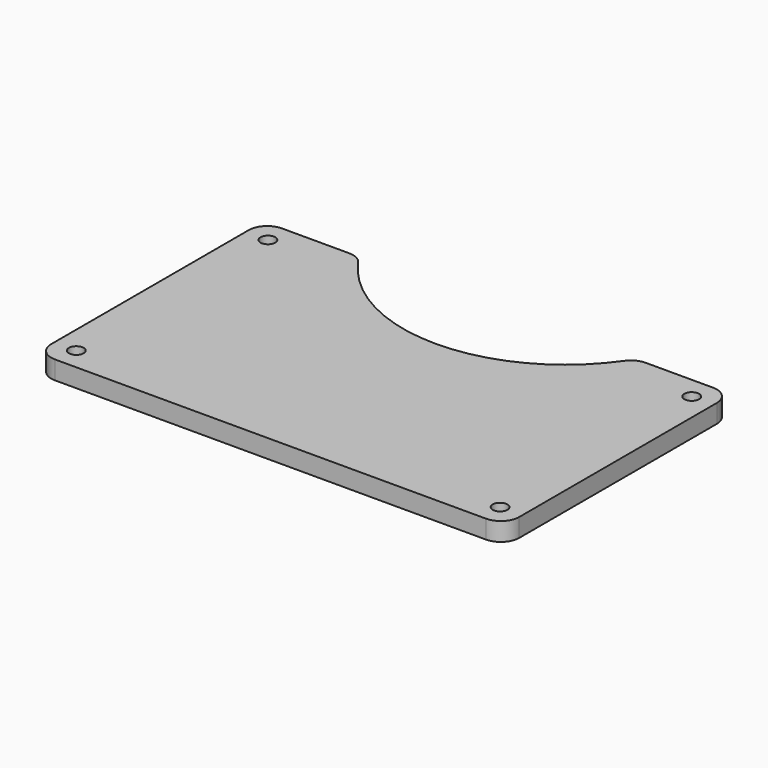
from build123d import *

# Parameters (mm, degrees)
F0_R     = 2
F1_DEPTH = 5
F2_R     = 3
F3_DEPTH = 0.6
F5_DEPTH = 2
F6_R     = 10
F7_R     = 2.5


with BuildPart() as f1:
    # F0 (on Top) → F1 (new body)
    with BuildSketch(Plane.XY):
        with BuildLine():
            Line((-58.5, -38.5), (58.5, -38.5))
            ThreePointArc((58.5, -38.5), (62.0355339059, -37.0355339059), (63.5, -33.5))
            Line((63.5, -33.5), (63.5, 33.5))
            ThreePointArc((63.5, 33.5), (62.0355339059, 37.0355339059), (58.5, 38.5))
            Line((58.5, 38.5), (40.2026118555, 38.5))
            ThreePointArc((40.2026118555, 38.5), (37.8876397432, 37.9318059659), (36.0988089683, 36.3563616478))
            ThreePointArc((36.0988089683, 36.3563616478), (0, 17.5), (-36.0988089683, 36.3563616478))
            ThreePointArc((-36.0988089683, 36.3563616478), (-37.8876397432, 37.9318059659), (-40.2026118555, 38.5))
            Line((-40.2026118555, 38.5), (-58.5, 38.5))
            ThreePointArc((-58.5, 38.5), (-62.0355339059, 37.0355339059), (-63.5, 33.5))
            Line((-63.5, 33.5), (-63.5, -33.5))
            ThreePointArc((-63.5, -33.5), (-62.0355339059, -37.0355339059), (-58.5, -38.5))
        make_face()
        with Locations((-57.5, -32.5)):
            Circle(F0_R, mode=Mode.SUBTRACT)
        with Locations((57.5, -32.5)):
            Circle(F0_R, mode=Mode.SUBTRACT)
        with Locations((-57.5, 32.5)):
            Circle(F0_R, mode=Mode.SUBTRACT)
        with Locations((57.5, 32.5)):
            Circle(F0_R, mode=Mode.SUBTRACT)
    extrude(amount=F1_DEPTH)

    # F2 (on face) → F3 (cut)
    with BuildSketch(Plane(origin=(0, 0, 0), x_dir=(1, 0, 0), z_dir=(0, 0, -1))):
        with Locations((-57.5, 32.5)):
            Circle(F2_R)
        with Locations((57.5, 32.5)):
            Circle(F2_R)
        with Locations((57.5, -32.5)):
            Circle(F2_R)
        with Locations((-57.5, -32.5)):
            Circle(F2_R)
    extrude(amount=-F3_DEPTH, mode=Mode.SUBTRACT)

    # F4 (on face) → F5 (cut)
    with BuildSketch(Plane(origin=(0, 0, 0), x_dir=(1, 0, 0), z_dir=(0, 0, -1))):
        Polygon((-8.542372966, 0), (-57.5000000613, 26.5), (-57.5, -26.5), align=None)
        Polygon((-4.0665, 32.5000000613), (-51.5, 32.5000000613), (-4.0665, 6.8249862876), align=None)
        Polygon((51.5, 32.5000000613), (4.0665, 32.5000000613), (4.0665, 6.8249862876), align=None)
        Polygon((57.5000000613, 26.5), (8.542372966, 0), (57.5000000613, -26.5), align=None)
    extrude(amount=-F5_DEPTH, mode=Mode.SUBTRACT)

    # F6
    f6_edges = [f1.edges().sort_by_distance(p)[0] for p in [
        (8.542373, 0, 1),
        (-8.542373, 0, 1),
        (-4.0665, -6.824986, 1),
        (4.0665, -6.824986, 1),
    ]]
    fillet(f6_edges, radius=F6_R)

    # F7
    f7_edges = [f1.edges().sort_by_distance(p)[0] for p in [
        (-51.5, -32.5, 1),
        (51.5, -32.5, 1),
        (57.5, -26.5, 1),
        (57.5, 26.5, 1),
        (-57.5, 26.5, 1),
        (-57.5, -26.5, 1),
        (4.0665, -32.5, 1),
        (-4.0665, -32.5, 1),
    ]]
    fillet(f7_edges, radius=F7_R)


solid = f1.part
